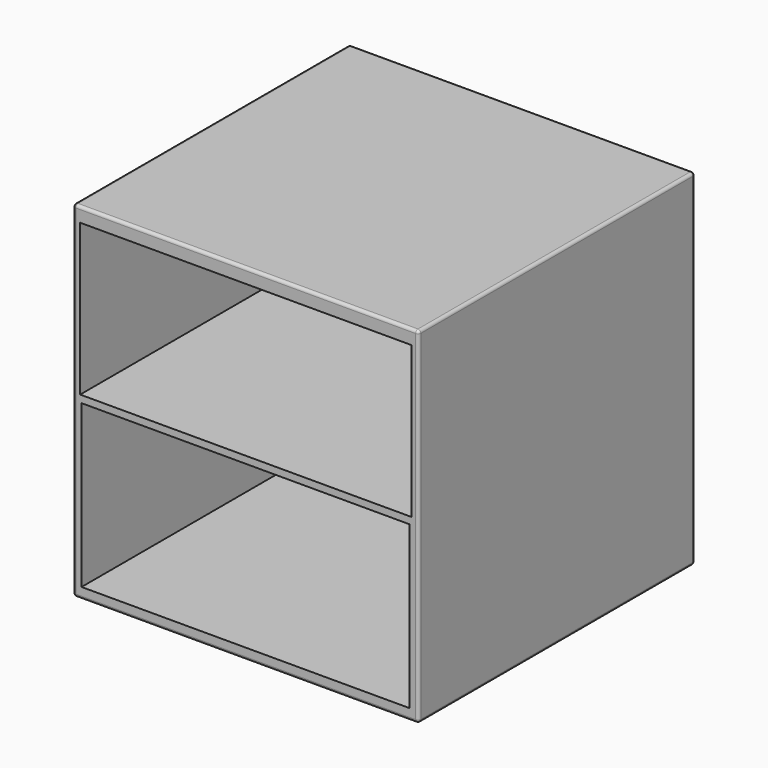
from build123d import *

# Parameters (mm, degrees)
F0_W         = 609.6
F0_H         = 609.6
F1_DEPTH     = 609.6
F3_R         = 5.08
F4_R         = 5.08
F5_T1_DEPTH  = 599.44
F5_T3_DEPTH  = 599.44
F5_T5_DEPTH  = 599.44
F5_S9_W      = 5.08
F5_S9_H      = 5.08
F5_T10_DEPTH = 5.08
F5_S15_W     = 5.08
F5_S15_H     = 5.08
F5_T16_DEPTH = 5.08
F5_S21_W     = 5.08
F5_S21_H     = 5.08
F5_T22_DEPTH = 5.08
F5_S27_W     = 5.08
F5_S27_H     = 5.08
F5_T28_DEPTH = 5.08
F5_T32_ANGLE = 90
F5_T34_ANGLE = 90
F2_W         = 584.2
F2_H         = 266.8860325682
F6_DEPTH     = 596.9
F7_W         = 578.0983269215
F7_H         = 285.4733169079
F8_DEPTH     = 596.9


# Not quite as in the source:
# - a fillet or chamfer that OpenCascade refuses, or shapes differently, is made with other operations: its cross-section is extruded or revolved along the edge and cut away or added


with BuildPart() as f1:
    # F0 (on Front) → F1 (new body)
    with BuildSketch(Plane.XZ):
        Rectangle(F0_W, F0_H)
    extrude(amount=F1_DEPTH)

    # F3
    f3_edges = [f1.edges().sort_by_distance(p)[0] for p in [
        (0, -609.6, 304.8),
    ]]
    fillet(f3_edges, radius=F3_R)

    # F4
    f4_edges = [f1.edges().sort_by_distance(p)[0] for p in [
        (-304.8, -609.6, -2.54),
        (304.8, -609.6, -2.54),
        (0, -609.6, -304.8),
    ]]
    fillet(f4_edges, radius=F4_R)

    # F5: fillet of radius 5.08 on 7 edges, made by hand

    # F5_s2 → F5_t1 (cut)
    with BuildSketch(Plane.XZ.offset(5.08)):
        with BuildLine():
            ThreePointArc((304.8, -299.72), (303.3121024484, -303.3121024484), (299.72, -304.8))
            Line((299.72, -304.8), (304.8, -304.8))
            Line((304.8, -304.8), (304.8, -299.72))
        make_face()
        with BuildLine():
            ThreePointArc((-304.8, -299.72), (-303.3121024484, -303.3121024484), (-299.72, -304.8))
            Line((-299.72, -304.8), (-304.8, -304.8))
            Line((-304.8, -304.8), (-304.8, -299.72))
        make_face()
    extrude(amount=F5_T1_DEPTH, mode=Mode.SUBTRACT)

    # F5_s4 → F5_t3 (cut)
    with BuildSketch(Plane.XY.offset(-299.72)):
        with BuildLine():
            ThreePointArc((299.72, 0), (303.3121024484, -1.4878975516), (304.8, -5.08))
            Line((304.8, -5.08), (304.8, 0))
            Line((304.8, 0), (299.72, 0))
        make_face()
        with BuildLine():
            ThreePointArc((-299.72, 0), (-303.3121024484, -1.4878975516), (-304.8, -5.08))
            Line((-304.8, -5.08), (-304.8, 0))
            Line((-304.8, 0), (-299.72, 0))
        make_face()
    extrude(amount=F5_T3_DEPTH, mode=Mode.SUBTRACT)

    # F5_s6 → F5_t5 (cut)
    with BuildSketch(Plane.YZ.offset(-299.72)):
        with BuildLine():
            ThreePointArc((-5.08, 304.8), (-1.4878975516, 303.3121024484), (0, 299.72))
            Line((0, 299.72), (0, 304.8))
            Line((0, 304.8), (-5.08, 304.8))
        make_face()
        with BuildLine():
            ThreePointArc((0, -299.72), (-1.4878975516, -303.3121024484), (-5.08, -304.8))
            Line((-5.08, -304.8), (0, -304.8))
            Line((0, -304.8), (0, -299.72))
        make_face()
    extrude(amount=F5_T5_DEPTH, mode=Mode.SUBTRACT)


with BuildPart() as f5_tool8:
    # F5_s9 → F5_t10 (new body)
    with BuildSketch(Plane.YZ.offset(-299.72)):
        with Locations((-607.06, -302.26)):
            Rectangle(F5_S9_W, F5_S9_H)
    extrude(amount=-F5_T10_DEPTH)

    # F5_s11 → F5_t12 (revolve, cut)
    with BuildSketch(Plane(origin=(-299.72, -604.52, -299.72), x_dir=(0, 0.7071067812, 0.7071067812), z_dir=(0, -0.7071067812, 0.7071067812))):
        with BuildLine():
            ThreePointArc((0, -5.08), (5.08, 0), (0, 5.08))
            Line((0, 5.08), (0, -5.08))
        make_face()
    revolve(axis=Axis((-299.72, -604.52, -299.72), (-1, 0, 0)), mode=Mode.SUBTRACT)


with BuildPart() as f1_1:
    add(f1.part)

    # F5_t7: cut F5_tool8
    add(f5_tool8.part, mode=Mode.SUBTRACT)


with BuildPart() as f5_tool14:
    # F5_s15 → F5_t16 (new body)
    with BuildSketch(Plane.YZ.offset(299.72)):
        with Locations((-607.06, -302.26)):
            Rectangle(F5_S15_W, F5_S15_H)
    extrude(amount=F5_T16_DEPTH)

    # F5_s17 → F5_t18 (revolve, cut)
    with BuildSketch(Plane(origin=(299.72, -604.52, -299.72), x_dir=(0, 0.7071067812, 0.7071067812), z_dir=(0, 0.7071067812, -0.7071067812))):
        with BuildLine():
            ThreePointArc((0, -5.08), (5.08, 0), (0, 5.08))
            Line((0, 5.08), (0, -5.08))
        make_face()
    revolve(axis=Axis((299.72, -604.52, -299.72), (1, 0, 0)), mode=Mode.SUBTRACT)


with BuildPart() as f1_2:
    add(f1_1.part)

    # F5_t13: cut F5_tool14
    add(f5_tool14.part, mode=Mode.SUBTRACT)


with BuildPart() as f5_tool20:
    # F5_s21 → F5_t22 (new body)
    with BuildSketch(Plane.YZ.offset(299.72)):
        with Locations((-2.54, -302.26)):
            Rectangle(F5_S21_W, F5_S21_H)
    extrude(amount=F5_T22_DEPTH)

    # F5_s23 → F5_t24 (revolve, cut)
    with BuildSketch(Plane(origin=(299.72, -5.08, -299.72), x_dir=(0, -0.7071067812, 0.7071067812), z_dir=(0, 0.7071067812, 0.7071067812))):
        with BuildLine():
            ThreePointArc((0, -5.08), (5.08, 0), (0, 5.08))
            Line((0, 5.08), (0, -5.08))
        make_face()
    revolve(axis=Axis((299.72, -5.08, -299.72), (1, 0, 0)), mode=Mode.SUBTRACT)


with BuildPart() as f1_3:
    add(f1_2.part)

    # F5_t19: cut F5_tool20
    add(f5_tool20.part, mode=Mode.SUBTRACT)


with BuildPart() as f5_tool26:
    # F5_s27 → F5_t28 (new body)
    with BuildSketch(Plane.YZ.offset(-299.72)):
        with Locations((-2.54, -302.26)):
            Rectangle(F5_S27_W, F5_S27_H)
    extrude(amount=-F5_T28_DEPTH)

    # F5_s29 → F5_t30 (revolve, cut)
    with BuildSketch(Plane(origin=(-299.72, -5.08, -299.72), x_dir=(0, -0.7071067812, 0.7071067812), z_dir=(0, -0.7071067812, -0.7071067812))):
        with BuildLine():
            ThreePointArc((0, -5.08), (5.08, 0), (0, 5.08))
            Line((0, 5.08), (0, -5.08))
        make_face()
    revolve(axis=Axis((-299.72, -5.08, -299.72), (-1, 0, 0)), mode=Mode.SUBTRACT)


with BuildPart() as f1_4:
    add(f1_3.part)

    # F5_t25: cut F5_tool26
    add(f5_tool26.part, mode=Mode.SUBTRACT)

    # F5_s31 → F5_t32 (revolve, cut)
    with BuildSketch(Plane.XY.offset(299.72)):
        with BuildLine():
            ThreePointArc((-304.8, -5.08), (-303.3121024484, -1.4878975516), (-299.72, 0))
            Line((-299.72, 0), (-304.8, 0))
            Line((-304.8, 0), (-304.8, -5.08))
        make_face()
    revolve(axis=Axis((-299.72, 0, 299.72), (0, 1, 0)), revolution_arc=F5_T32_ANGLE, mode=Mode.SUBTRACT)

    # F5_s33 → F5_t34 (revolve, cut)
    with BuildSketch(Plane.XY.offset(299.72)):
        with BuildLine():
            ThreePointArc((304.8, -5.08), (303.3121024484, -1.4878975516), (299.72, 0))
            Line((299.72, 0), (304.8, 0))
            Line((304.8, 0), (304.8, -5.08))
        make_face()
    revolve(axis=Axis((299.72, 0, 299.72), (0, -1, 0)), revolution_arc=F5_T34_ANGLE, mode=Mode.SUBTRACT)

    # F2 (on face) → F6 (cut)
    with BuildSketch(Plane.XZ.offset(609.6)):
        with Locations((0, 145.9569837159)):
            Rectangle(F2_W, F2_H)
    extrude(amount=-F6_DEPTH, mode=Mode.SUBTRACT)

    # F7 (on face) → F8 (cut)
    with BuildSketch(Plane.XZ.offset(609.6)):
        with Locations((-0.5959719419, -142.7366584539)):
            Rectangle(F7_W, F7_H)
    extrude(amount=-F8_DEPTH, mode=Mode.SUBTRACT)


solid = f1_4.part
